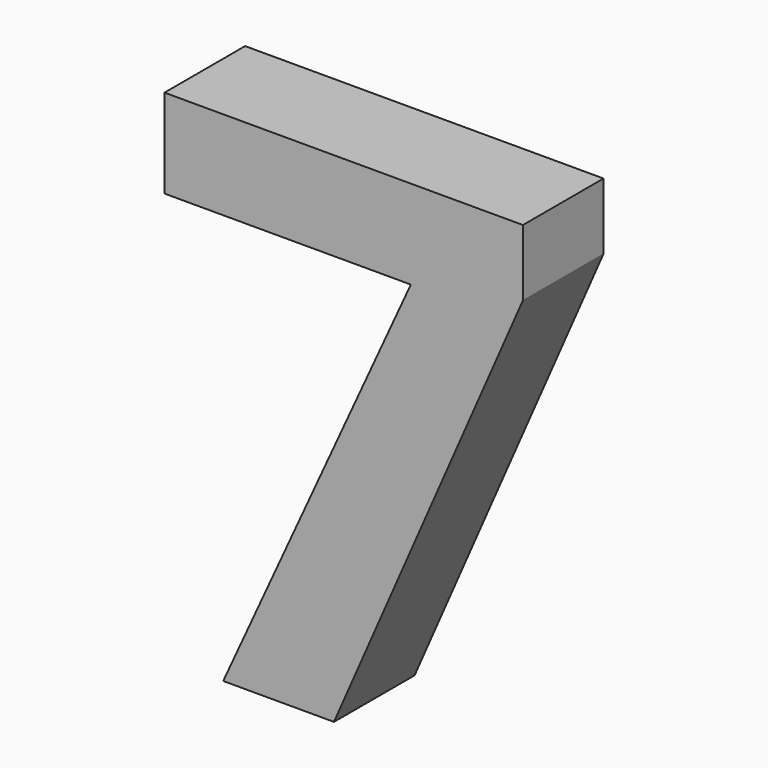
from build123d import *

# Parameters (mm, degrees)
F0_TEXT_SIZE = 35.2777777778
F1_DEPTH     = 5.08


# Not quite as in the source:
# - Text() gives the source's letters only with a copy of the font that has no kerning and outlines rounded to 1/6400 em; it was checked with that copy


with BuildPart() as f1:
    # F0 (on Front) → F1 (new body)
    with BuildSketch(Plane.XZ):
        with Locations((-22.0474900621, -2.3679110635)):
            Text('7', F0_TEXT_SIZE, font='Open Sans', font_style=FontStyle.BOLD, text_align=(TextAlign.LEFT, TextAlign.BOTTOM))
    extrude(amount=F1_DEPTH)


solid = f1.part
